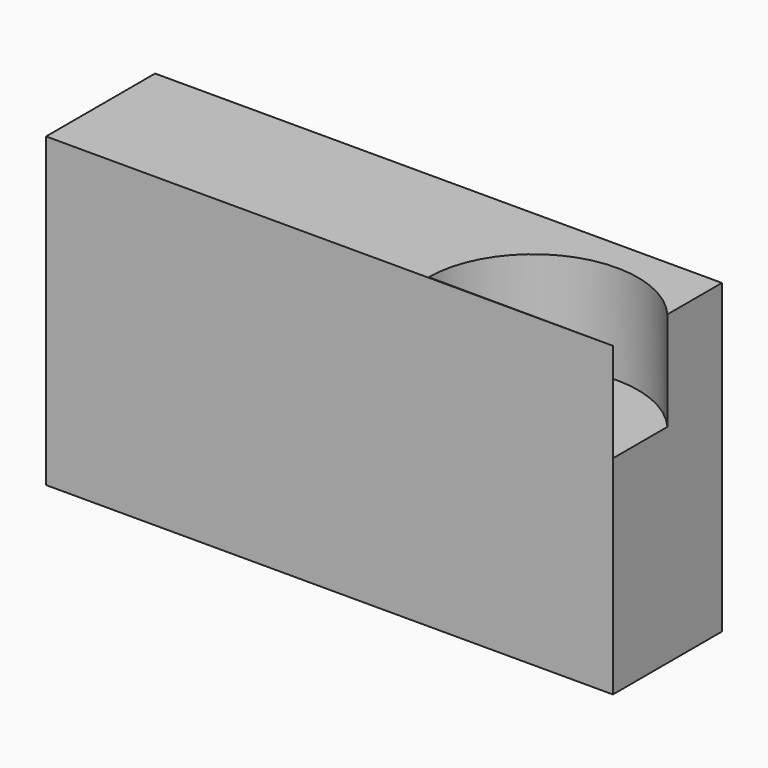
from build123d import *

# Parameters (mm, degrees)
F0_W     = 145.4039812088
F0_H     = 34.9461883307
F1_DEPTH = 78.74
F5_DEPTH = 25.4


# Not quite as in the source:
# - the program builds the solid bodies; features that only make, move or delete a surface that nothing else refers to are left out


with BuildPart() as f1:
    # F0 (on Top) → F1 (new body)
    with BuildSketch(Plane.XY):
        with Locations((72.7019906044, 72.0167830586)):
            Rectangle(F0_W, F0_H)
    extrude(amount=F1_DEPTH)

    # F4 (on face) → F5 (cut)
    with BuildSketch(Plane.XY.offset(78.74)):
        with BuildLine():
            Line((145.4039812088, 54.5436888933), (145.4039812088, 72.0167830586))
            ThreePointArc((145.4039812088, 72.0167830586), (115.6911009346, 79.8555366854), (97.9683505694, 54.7516439176))
            Line((97.9683505694, 54.7516439176), (145.4039812088, 54.5436888933))
        make_face()
    extrude(amount=-F5_DEPTH, mode=Mode.SUBTRACT)


solid = f1.part
